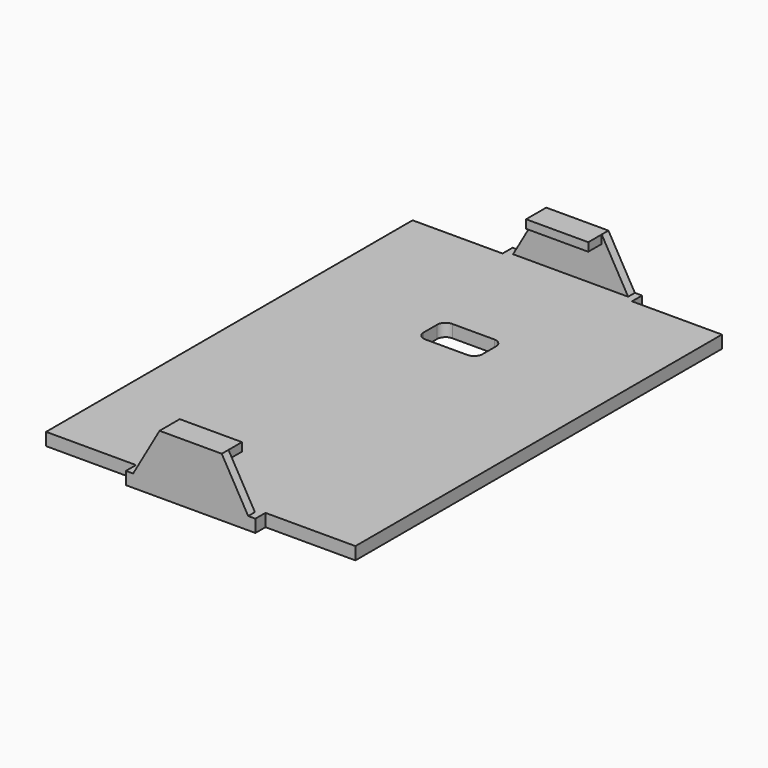
from build123d import *

# Parameters (mm, degrees)
F0_W     = 7
F0_H     = 4
F0_W_2   = 15.4
F0_H_2   = 0.5
F1_DEPTH = 1.5
F2_W     = 7.4
F2_H     = 1.5
F2_H_2   = 4.5
F2_H_3   = 1
F3_DEPTH = 1
F4_DEPTH = 2
F6_R     = 1


with BuildPart() as f1:
    # F0 (on Top) → F1 (new body)
    with BuildSketch(Plane.XY):
        Polygon((7.7, -27.25), (18.4, -27.25), (18.4, 27.25), (7.7, 27.25), (-7.7, 27.25), (-18.4, 27.25), (-18.4, -27.25), (-7.7, -27.25), align=None)
        with Locations((0, 11.2744159997)):
            Rectangle(F0_W, F0_H, mode=Mode.SUBTRACT)
        with Locations((0, -27.5)):
            Rectangle(F0_W_2, F0_H_2)
        with Locations((0, 27.5)):
            Rectangle(F0_W_2, F0_H_2)
    extrude(amount=F1_DEPTH)



with BuildPart() as f3:
    # F2 (on face) → F3 (new body)
    with BuildSketch(Plane.XZ.offset(27.75)):
        Polygon((-7.7, 0), (-3.7, 0), (-3.7, 1.5), (-6.8428571429, 1.5), align=None)
        with Locations((0, 0.75)):
            Rectangle(F2_W, F2_H)
        Polygon((3.7, 1.5), (3.7, 0), (7.7, 0), (6.8428571429, 1.5), align=None)
        Polygon((-6.8428571429, 1.5), (-3.7, 1.5), (-3.7, 6), (-3.7, 7), align=None)
        with Locations((0, 3.75)):
            Rectangle(F2_W, F2_H_2)
        with Locations((0, 6.5)):
            Rectangle(F2_W, F2_H_3)
        Polygon((3.7, 6), (3.7, 1.5), (6.8428571429, 1.5), (3.7, 7), align=None)
        Polygon((6.8428571429, 1.5), (7.7, 0), (7.7, 1.5), align=None)
        Polygon((-7.7, 1.5), (-7.7, 0), (-6.8428571429, 1.5), align=None)
    extrude(amount=F3_DEPTH)


with BuildPart() as f4:
    # F2 (on face) → F4 (new body)
    with BuildSketch(Plane.XZ.offset(27.75)):
        with Locations((0, 6.5)):
            Rectangle(F2_W, F2_H_3)
    extrude(amount=-F4_DEPTH)


with BuildPart() as f1_1:
    add(f1.part)

    add(f3.part)  # F5 merges F3

    add(f4.part)  # F5 merges F4
    # F5: F3, F4 across plane
    add(f3.part.mirror(Plane.XZ))
    add(f4.part.mirror(Plane.XZ))

    # F6
    f6_edges = [f1_1.edges().sort_by_distance(p)[0] for p in [
        (-3.5, 13.274416, 0.75),
        (-3.5, 9.274416, 0.75),
        (3.5, 9.274416, 0.75),
        (3.5, 13.274416, 0.75),
    ]]
    fillet(f6_edges, radius=F6_R)


solid = f1_1.part
